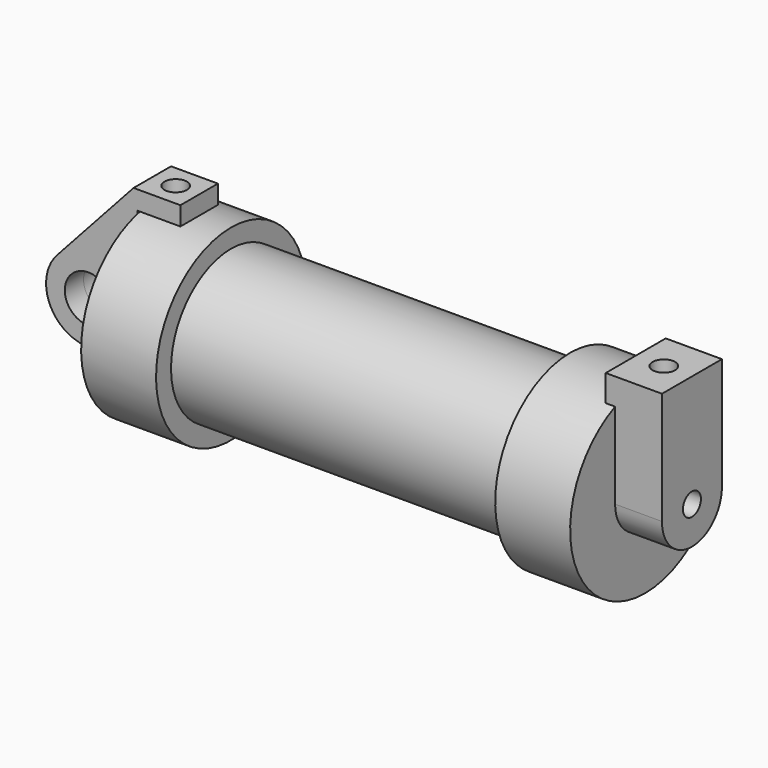
from build123d import *

# Parameters (mm, degrees)
F0_W          = 5.842
F0_H          = 12.7
F2_DEPTH      = 3.175
F2_DEPTH_BACK = 3.175
F0_R          = 3.175
F3_DEPTH      = 3.175
F3_DEPTH_BACK = 3.175
F4_R          = 1.524
F5_DEPTH      = 6.35
F5_DEPTH_BACK = 1.27
F6_DEPTH      = 56.134
F7_R          = 1.524
F8_DEPTH      = 17.78
F9_R          = 1.524
F10_DEPTH     = 10.414


with BuildPart() as f1:
    # F0 (on Front) → F1 (revolve)
    with BuildSketch(Plane.XZ):
        with Locations((2.921, 6.35)):
            Rectangle(F0_W, F0_H)
        Polygon((5.842, 12.7), (5.842, 0), (66.294, 0), (66.294, 12.7), (56.134, 12.7), (56.134, 10.16), (10.16, 10.16), (10.16, 12.7), align=None)
    revolve(axis=Axis((-3.3274, 0, 0), (-1, 0, 0)))

    # F4 (on face) → F5 (join, two sides)
    with BuildSketch(Plane.YZ.offset(66.294)) as f5_sk:
        with BuildLine():
            ThreePointArc((-5.08, 0), (0, -5.08), (5.08, 0))
            ThreePointArc((5.08, 0), (0, 5.08), (-5.08, 0))
        make_face()
        Circle(F4_R, mode=Mode.SUBTRACT)
        with BuildLine():
            ThreePointArc((-5.08, 0), (0, 5.08), (5.08, 0))
            Line((5.08, 0), (5.08, 15.24))
            Line((5.08, 15.24), (-5.08, 15.24))
            Line((-5.08, 15.24), (-5.08, 0))
        make_face()
    extrude(amount=F5_DEPTH)
    extrude(f5_sk.sketch, amount=-F5_DEPTH_BACK)

    # F6 (cut, through all): a face of the model
    f6_faces = [f1.faces().sort_by_distance(p)[0] for p in [
        (66.294, 0, 0),
    ]]
    extrude(f6_faces, amount=-F6_DEPTH, mode=Mode.SUBTRACT)

    # F9 (on face) → F10 (cut)
    with BuildSketch(Plane.XY.offset(15.24)):
        with Locations((68.834, 0)):
            Circle(F9_R)
    extrude(amount=-F10_DEPTH, mode=Mode.SUBTRACT)


with BuildPart() as f2:
    # F0 (on Front) → F2 (new body, two sides)
    with BuildSketch(Plane.XZ) as f2_sk:
        with BuildLine():
            Line((-0.9398, 0), (0, 0))
            Line((0, 0), (0, 12.7))
            Line((0, 12.7), (5.842, 12.7))
            Line((5.842, 12.7), (5.842, 15.24))
            Line((5.842, 15.24), (-0.508, 15.24))
            Line((-0.508, 15.24), (-10.8806298187, 3.8475430269))
            ThreePointArc((-10.8806298187, 3.8475430269), (-4.5919612295, 5.3297205562), (-0.9398, 0))
        make_face()
        with BuildLine():
            Line((5.842, 0), (0, 0))
            Line((0, 0), (-0.9398, 0))
            ThreePointArc((-0.9398, 0), (-3.1957909266, -4.5493385486), (-8.1826630726, -5.5069827884))
            Line((-8.1826630726, -5.5069827884), (5.842, -9.398))
            Line((5.842, -9.398), (5.842, 0))
        make_face()
    extrude(amount=F2_DEPTH)
    extrude(f2_sk.sketch, amount=-F2_DEPTH_BACK)

    # F0 (on Front) → F3 (join, two sides)
    with BuildSketch(Plane.XZ) as f3_sk:
        with BuildLine():
            ThreePointArc((-8.1826630726, -5.5069827884), (-3.1957909266, -4.5493385486), (-0.9398, 0))
            ThreePointArc((-0.9398, 0), (-4.5919612295, 5.3297205562), (-10.8806298187, 3.8475430269))
            ThreePointArc((-10.8806298187, 3.8475430269), (-12.1459778134, -1.5837270034), (-8.1826630726, -5.5069827884))
        make_face()
        with Locations((-6.6548, 0)):
            Circle(F0_R, mode=Mode.SUBTRACT)
    extrude(amount=F3_DEPTH)
    extrude(f3_sk.sketch, amount=-F3_DEPTH_BACK)

    # F7 (on face) → F8 (cut)
    with BuildSketch(Plane.XY.offset(15.24)):
        with Locations((2.667, 0)):
            Circle(F7_R)
    extrude(amount=-F8_DEPTH, mode=Mode.SUBTRACT)


solid = Compound([f1.part, f2.part])
